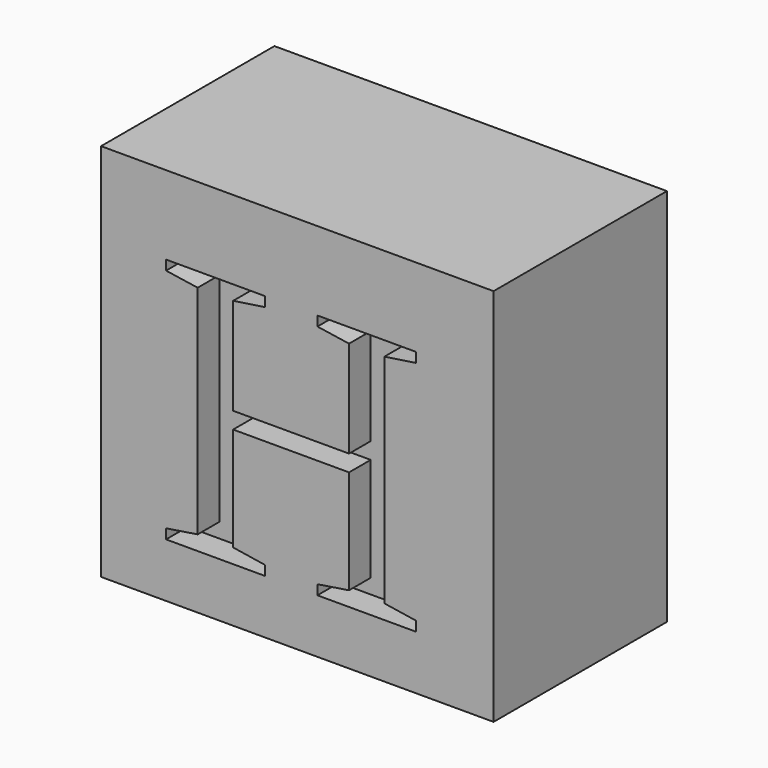
from build123d import *

# Parameters (mm, degrees)
F1_W         = 46.0071841015
F1_H         = 44.4500009418
F2_DEPTH     = 25.4
F0_TEXT_SIZE = 44.0972222222
F3_DEPTH     = 3.175


# Not quite as in the source:
# - Text() gives the source's letters only with a copy of the font that has no kerning and outlines rounded to 1/6400 em; it was checked with that copy


with BuildPart() as f2:
    # F1 (on Front) → F2 (new body)
    with BuildSketch(Plane.XZ):
        with Locations((16.6535915799, 15.875)):
            Rectangle(F1_W, F1_H)
    extrude(amount=-F2_DEPTH)

    # F0 (on Front) → F3 (cut)
    with BuildSketch(Plane.XZ):
        with Locations((0, 0)):
            Text('H', F0_TEXT_SIZE, font='Tinos', text_align=(TextAlign.LEFT, TextAlign.BOTTOM))
    extrude(amount=-F3_DEPTH, mode=Mode.SUBTRACT)


solid = f2.part
